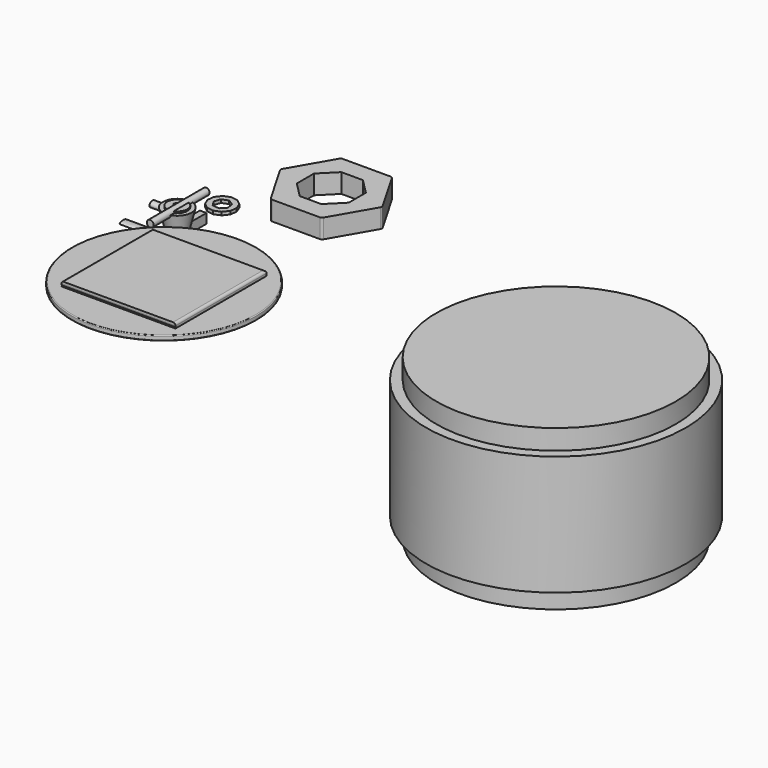
from build123d import *

# Parameters (mm, degrees)
F1_DEPTH  = 25.4
F3_DEPTH  = 51.308
F5_DEPTH  = 305.1048
F6_R      = 45.72
F7_R      = 1465.0405111475
F7_W      = 1814.1152858734
F7_H      = 1814.1152858734
F8_DEPTH  = 76.2
F9_DEPTH  = 76.2
F10_R     = 38.09999
F11_R     = 12.7
F12_R     = 1905
F13_DEPTH = 1270
F12_R_2   = 2063.75
F14_DEPTH = 952.5
F19_R     = 229.0809109199
F21_R     = 154.6394893279
F23_W     = 104.8123165965
F23_H     = 816.8393224478
F24_DEPTH = 76.2
F26_DEPTH = 643.5099393129
F27_R     = 53.8997804339
F28_DEPTH = 556.3534796238


# Not quite as in the source:
# - a fillet or chamfer is up to 0.001 mm smaller than in the source, because OpenCascade refuses the exact size
# - the program builds the solid bodies; features that only make, move or delete a surface that nothing else refers to are left out


with BuildPart() as f1:
    # F0 (on Top) → F1 (new body)
    with BuildSketch(Plane.XY):
        Polygon((155.50936864, 47.9948012801), (122.5436329842, 107.0967912674), (68.3889899114, 147.6807731007), (2.4092691885, 162.7294076272), (-63.9870360646, 149.6406492247), (-119.3194014782, 110.6776631286), (-154.0203583934, 52.5775036026), (-162.0897961115, -14.6137839479), (-142.1324355422, -79.2782154918), (-97.5990856351, -130.2347233572), (-36.1899671618, -158.6724644088), (31.4767254093, -159.67429487), (93.7008062, -133.0669891528), (139.7231663537, -83.4511921354), (161.5861216997, -19.4059258675), align=None)
        Polygon((39.7706934855, 64.0896567419), (63.5851919651, 21.2782472372), (50.1523473576, -25.8333841012), (7.3409378529, -49.6478825808), (-39.7706934855, -36.2150379733), (-63.5851919651, 6.5963715315), (-50.1523473576, 53.7080028699), (-7.3409378529, 77.5225013494), align=None, mode=Mode.SUBTRACT)
    extrude(amount=F1_DEPTH)


with BuildPart() as f3:
    # F2 (on Top) → F3 (new body)
    with BuildSketch(Plane.XY):
        Polygon((567.1581641405, 172.1189159194), (635.2695226669, 258.6906254292), (650.9698346822, 367.7196043769), (610.052214261, 469.9916259019), (523.4805047512, 538.1029844284), (414.4515258035, 553.8032964437), (312.1795042784, 512.8856760224), (244.068145752, 426.3139665127), (228.3678337366, 317.284987565), (269.2854541579, 215.0129660399), (355.8571636677, 146.9016075134), (464.8861426154, 131.2012954981), align=None)
        Polygon((545.1443835194, 410.1638138472), (558.3316683769, 302.2244572639), (482.1634188256, 224.6151347452), (373.9958803268, 235.7772490893), (315.2814155857, 327.3055005294), (350.2332141092, 430.2772488952), (452.5318587224, 467.1526674262), align=None, mode=Mode.SUBTRACT)
    extrude(amount=F3_DEPTH)


with BuildPart() as f5:
    # F4 (on Top) → F5 (new body)
    with BuildSketch(Plane.XY):
        Polygon((1943.6769121667, 437.2407213386), (2349.1595144473, 1139.5571900737), (1943.6769121667, 1841.8736588088), (1132.7117076057, 1841.8736588088), (727.2291053252, 1139.5571900737), (1132.7117076057, 437.2407213386), align=None)
        Polygon((1709.2926557119, 1552.6251370658), (1951.2622568783, 1310.6555358994), (1951.2622568783, 968.458844248), (1709.2926557119, 726.4892430816), (1367.0959640605, 726.4892430816), (1125.1263628941, 968.458844248), (1125.1263628941, 1310.6555358994), (1367.0959640605, 1552.6251370658), align=None, mode=Mode.SUBTRACT)
    extrude(amount=F5_DEPTH)

    # F6
    f6_edges = [f5.edges().sort_by_distance(p)[0] for p in [
        (1943.676912, 437.240721, 152.5524),
        (2349.159514, 1139.55719, 152.5524),
        (1943.676912, 1841.873659, 152.5524),
        (1132.711708, 1841.873659, 152.5524),
        (727.229105, 1139.55719, 152.5524),
        (1132.711708, 437.240721, 152.5524),
    ]]
    fillet(f6_edges, radius=F6_R)


with BuildPart() as f8:
    # F7 (on Top) → F8 (new body)
    with BuildSketch(Plane.XY):
        with Locations((1112.9351854324, -1654.5432806015)):
            Circle(F7_R)
        with Locations((1112.9351854324, -1654.5432806015)):
            Rectangle(F7_W, F7_H, mode=Mode.SUBTRACT)
    extrude(amount=-F8_DEPTH)

    # F11
    f11_edges = [f8.edges().sort_by_distance(p)[0] for p in [
        (-352.105326, -1654.543281, 0),
        (-352.105326, -1654.543281, -76.2),
    ]]
    fillet(f11_edges, radius=F11_R)


with BuildPart() as f9:
    # F7 (on Top) → F9 (new body)
    with BuildSketch(Plane.XY):
        with Locations((1112.9351854324, -1654.5432806015)):
            Rectangle(F7_W, F7_H)
    extrude(amount=F9_DEPTH)

    # F10 (radius 38.1 in the source; OpenCascade refuses exactly that, so slightly less here)
    f10_edges = [f9.edges().sort_by_distance(p)[0] for p in [
        (205.877542, -1654.543281, 76.2),
        (2019.992828, -1654.543281, 76.2),
        (1112.935185, -2561.600924, 0),
        (1112.935185, -747.485638, 76.2),
    ]]
    fillet(f10_edges, radius=F10_R)


with BuildPart() as f13:
    # F12 (on Top) → F13 (new body, symmetric)
    with BuildSketch(Plane.XY):
        with Locations((7716.8588638306, -2116.8828010559)):
            Circle(F12_R)
    extrude(amount=F13_DEPTH, both=True)

    # F12 (on Top) → F14 (join, symmetric)
    with BuildSketch(Plane.XY):
        with Locations((7716.8588638306, -2116.8828010559)):
            Circle(F12_R_2)
        with Locations((7716.8588638306, -2116.8828010559)):
            Circle(F12_R, mode=Mode.SUBTRACT)
    extrude(amount=F14_DEPTH, both=True)


with BuildPart() as f22:
    # F19 (on Top) → F22 section 0
    with BuildSketch(Plane.XY):
        Circle(F19_R)
    # F21 (on offset) → F22 section 1
    with BuildSketch(Plane.XY.offset(-304.8)):
        Circle(F21_R)
    loft()

    # F23 (on offset) → F24 (join, symmetric)
    with BuildSketch(Plane.XY.offset(-304.8)):
        with Locations((52.4061582983, 40.6319275498)):
            Rectangle(F23_W, F23_H)
    extrude(amount=F24_DEPTH, both=True)

    # F25 (on face) → F26 (join)
    with BuildSketch(Plane(origin=(0, 0, 0), x_dir=(0, -1, 0), z_dir=(-1, 0, 0))):
        with BuildLine():
            add(Edge.make_bspline(
                [(204.6898007393, -302.1550476551), (204.6898007393, -345.0046976312), (306.7133426666, -323.5798726431), (408.736884594, -302.1550476551), (306.7133426666, -280.7302226671), (204.6898007393, -259.305397679), (204.6898007393, -302.1550476551)],
                knots=[0, 0, 0, 2.0943951024, 2.0943951024, 4.1887902048, 4.1887902048, 6.2831853072, 6.2831853072, 6.2831853072], degree=2, weights=[1, 0.5, 1, 0.5, 1, 0.5, 1]))
        make_face()
        with BuildLine():
            add(Edge.make_bspline(
                [(-369.6652650833, -287.2584462166), (-369.6652650833, -367.9612465382), (-280.7216048241, -327.6098463774), (-191.7779445648, -287.2584462166), (-280.7216048241, -246.9070460558), (-369.6652650833, -206.555645895), (-369.6652650833, -287.2584462166)],
                knots=[0, 0, 0, 2.0943951024, 2.0943951024, 4.1887902048, 4.1887902048, 6.2831853072, 6.2831853072, 6.2831853072], degree=2, weights=[1, 0.5, 1, 0.5, 1, 0.5, 1]))
        make_face()
    extrude(amount=F26_DEPTH)

    # F27 (on Front) → F28 (join, symmetric)
    with BuildSketch(Plane.XZ):
        with Locations((14.3709331751, 0)):
            Circle(F27_R)
    extrude(amount=F28_DEPTH, both=True)


solid = Compound([f1.part, f3.part, f5.part, f8.part, f9.part, f13.part, f22.part])
